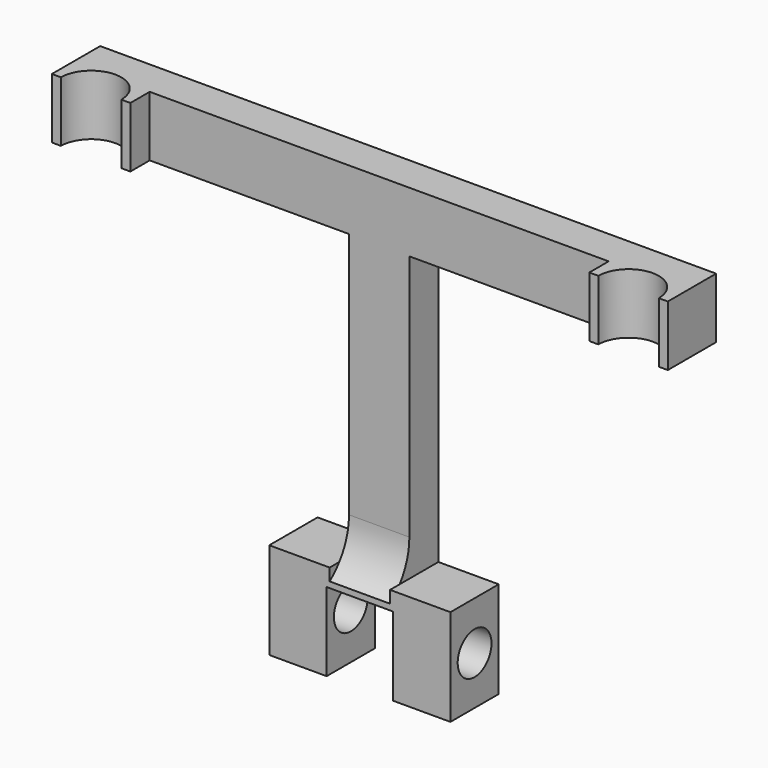
from build123d import *

# Parameters (mm, degrees)
F0_W        = 5
F0_H        = 2.5
F0_H_2      = 23.5
F0_H_3      = 4
F1_DEPTH    = 5
F2_W        = 5.5
F2_H        = 5.6794419712
F3_DEPTH    = 6.5
F4_R        = 1.75
F5_DEPTH    = 25.4
F6_W        = 5
F6_H        = 24.5096784085
F6_W_2      = 23
F6_H_2      = 5
F7_DEPTH    = 2
F8_T1_DEPTH = 5
F9_W        = 6.5
F9_H        = 5
F10_DEPTH   = 2
F11_R       = 2.5
F12_DEPTH   = 36.501


# Not quite as in the source:
# - a fillet or chamfer that OpenCascade refuses, or shapes differently, is made with other operations: its cross-section is extruded or revolved along the edge and cut away or added


with BuildPart() as f1:
    # F0 (on Front) → F1 (new body)
    with BuildSketch(Plane.XZ):
        with Locations((0, 13.75)):
            Rectangle(F0_W, F0_H)
        Polygon((-2.5, 15), (2.5, 15), (2.5, 12.5), (25.5, 12.5), (25.5, 17.5), (-25.5, 17.5), (-25.5, 12.5), (-2.5, 12.5), align=None)
        with Locations((0, 0.75)):
            Rectangle(F0_W, F0_H_2)
        Polygon((7.5, -11), (2.5, -11), (2.5, -15), (-2.5, -15), (-2.5, -11), (-7.5, -11), (-7.5, -19), (7.5, -19), align=None)
        with Locations((0, -13)):
            Rectangle(F0_W, F0_H_3)
    extrude(amount=F1_DEPTH)

    # F2 (on face) → F3 (cut)
    with BuildSketch(Plane(origin=(0, 0, -19), x_dir=(1, 0, 0), z_dir=(0, 0, -1))):
        with Locations((0, 2.1602790144)):
            Rectangle(F2_W, F2_H)
    extrude(amount=-F3_DEPTH, mode=Mode.SUBTRACT)

    # F4 (on face) → F5 (cut)
    with BuildSketch(Plane(origin=(-7.5, 0, 0), x_dir=(0, -1, 0), z_dir=(-1, 0, 0))):
        with Locations((2.5, -15)):
            Circle(F4_R)
    extrude(amount=-F5_DEPTH, mode=Mode.SUBTRACT)

    # F6 (on face) → F7 (cut)
    with BuildSketch(Plane.XZ.offset(5)):
        with Locations((0, 0.2451607957)):
            Rectangle(F6_W, F6_H)
        with Locations((-14, 15)):
            Rectangle(F6_W_2, F6_H_2)
        with Locations((0, 15)):
            Rectangle(F6_W, F6_H_2)
        with Locations((14, 15)):
            Rectangle(F6_W_2, F6_H_2)
    extrude(amount=-F7_DEPTH, mode=Mode.SUBTRACT)

    # F8: fillet of radius 5.08 on 1 edges, made by hand

    # F8_s2 → F8_t1 (join)
    with BuildSketch(Plane.YZ.offset(-2.5)):
        with BuildLine():
            ThreePointArc((-3, -7.9698764332), (-3.5273743839, -10.2237619671), (-5, -12.0096784085))
            Line((-5, -12.0096784085), (-3, -12.0096784085))
            Line((-3, -12.0096784085), (-3, -7.9698764332))
        make_face()
    extrude(amount=F8_T1_DEPTH)

    # F9 (on face) → F10 (join)
    with BuildSketch(Plane.XZ.offset(3)):
        with Locations((22.25, 15)):
            Rectangle(F9_W, F9_H)
        with Locations((-22.25, 15)):
            Rectangle(F9_W, F9_H)
    extrude(amount=F10_DEPTH)

    # F11 (on face) → F12 (cut, through all)
    with BuildSketch(Plane.XY.offset(17.5)):
        with Locations((22.25, -5)):
            Circle(F11_R)
        with Locations((-22.25, -5)):
            Circle(F11_R)
    extrude(amount=-F12_DEPTH, mode=Mode.SUBTRACT)


solid = f1.part
